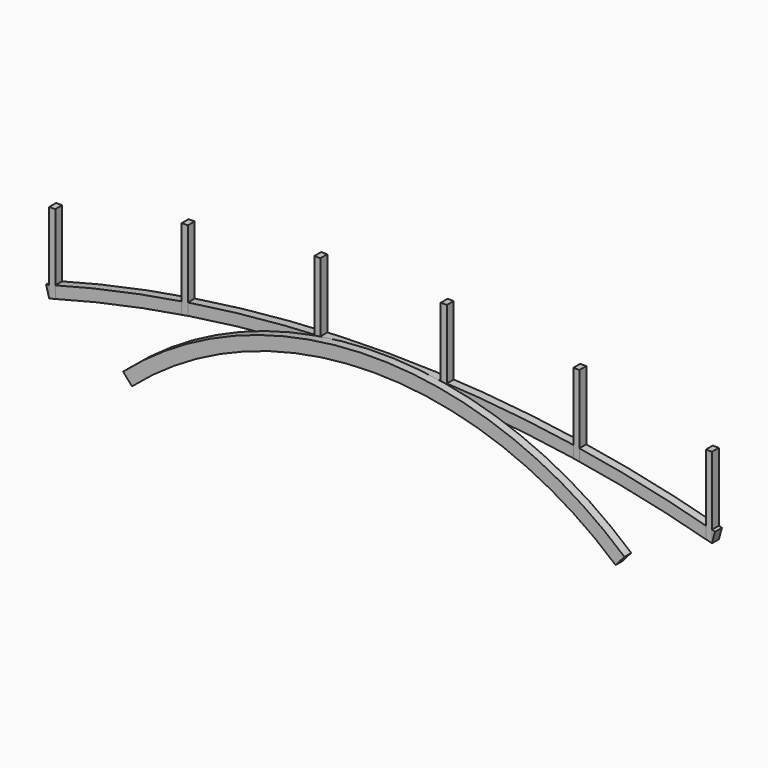
from build123d import *

# Parameters (mm, degrees)
F1_E7_W  = 150
F1_E7_H  = 95
F3_E9_W  = 130
F3_E9_H  = 96
F6_DEPTH = 96


with BuildPart() as f2:
    # F2: sweep along a path in F0
    with BuildLine(Plane.XZ) as f2_path:
        ThreePointArc((2028, -500), (-672, 514.5502758917), (-3372, -500))
    # F1_E7 (on explicit) → F2 (sweep)
    with BuildSketch(Plane(origin=(-3372, 0, -500), x_dir=(-0.6585365854, 0, 0.7525487132), z_dir=(0.7525487132, 0, 0.6585365854))):
        with Locations((75, 47.5)):
            Rectangle(F1_E7_W, F1_E7_H)
    sweep(path=f2_path.line)


with BuildPart() as f4:
    # F4: sweep along a path in F0
    with BuildLine(Plane.XZ) as f4_path:
        ThreePointArc((3028, 0), (-672, 500), (-4372, 0))
    # F3_E9 (on explicit) → F4 (sweep)
    with BuildSketch(Plane(origin=(-4372, 0, 0), x_dir=(-0.2654232425, 0, 0.9641319943), z_dir=(0.9641319943, 0, 0.2654232425))):
        with Locations((65, 48)):
            Rectangle(F3_E9_W, F3_E9_H)
    sweep(path=f4_path.line)


with BuildPart() as f4_1:
    # F5: moved
    add(f4.part.moved(Location((0, 96, 0))))


with BuildPart() as f6:
    # F0 (on Front) → F6 (new body)
    with BuildSketch(Plane.XZ):
        with BuildLine():
            Line((-4372, 900), (-4372, 0))
            ThreePointArc((-4372, 0), (-4338.0117144615, 9.3106927244), (-4304, 18.5354329511))
            Line((-4304, 18.5354329511), (-4304, 900))
            Line((-4304, 900), (-4372, 900))
        make_face()
    extrude(amount=-F6_DEPTH)


with BuildPart() as f6b:
    # F0 (on Front) → F6, piece 2 (new body)
    with BuildSketch(Plane.XZ):
        with BuildLine():
            Line((-2892, 1222.0928640959), (-2892, 322.0928640959))
            ThreePointArc((-2892, 322.0928640959), (-2858.0066660368, 327.5333613557), (-2824, 332.8898928293))
            Line((-2824, 332.8898928293), (-2824, 1222.0928640959))
            Line((-2824, 1222.0928640959), (-2892, 1222.0928640959))
        make_face()
    extrude(amount=-F6_DEPTH)


with BuildPart() as f6c:
    # F0 (on Front) → F6, piece 3 (new body)
    with BuildSketch(Plane.XZ):
        with BuildLine():
            ThreePointArc((-1412, 480.3448233153), (-1378.0021053501, 482.1105090874), (-1344, 483.793161348))
            Line((-1344, 483.793161348), (-1344, 1380.3448233153))
            Line((-1344, 1380.3448233153), (-1412, 1380.3448233153))
            Line((-1412, 1380.3448233153), (-1412, 480.3448233153))
        make_face()
    extrude(amount=-F6_DEPTH)


with BuildPart() as f6d:
    # F0 (on Front) → F6, piece 4 (new body)
    with BuildSketch(Plane.XZ):
        with BuildLine():
            Line((0, 1380.3448233152), (0, 483.793161348))
            ThreePointArc((0, 483.793161348), (34.0021053501, 482.1105090874), (68, 480.3448233153))
            Line((68, 480.3448233152), (68, 1380.3448233152))
            Line((68, 1380.3448233152), (0, 1380.3448233152))
        make_face()
    extrude(amount=-F6_DEPTH)


with BuildPart() as f6e:
    # F0 (on Front) → F6, piece 5 (new body)
    with BuildSketch(Plane.XZ):
        with BuildLine():
            ThreePointArc((1480, 332.8898928293), (1514.0066660368, 327.5333613557), (1548, 322.0928640959))
            Line((1548, 322.0928640959), (1548, 1222.0928640959))
            Line((1548, 1222.0928640959), (1480, 1222.0928640959))
            Line((1480, 1222.0928640959), (1480, 332.8898928293))
        make_face()
    extrude(amount=-F6_DEPTH)


with BuildPart() as f6f:
    # F0 (on Front) → F6, piece 6 (new body)
    with BuildSketch(Plane.XZ):
        with BuildLine():
            ThreePointArc((2960, 18.5354329511), (2994.0117144615, 9.3106927244), (3028, 0))
            Line((3028, 0), (3028, 900))
            Line((3028, 900), (2960, 900))
            Line((2960, 900), (2960, 18.5354329511))
        make_face()
    extrude(amount=-F6_DEPTH)


solid = Compound([f2.part, f4_1.part, f6.part, f6b.part, f6c.part, f6d.part, f6e.part, f6f.part])
